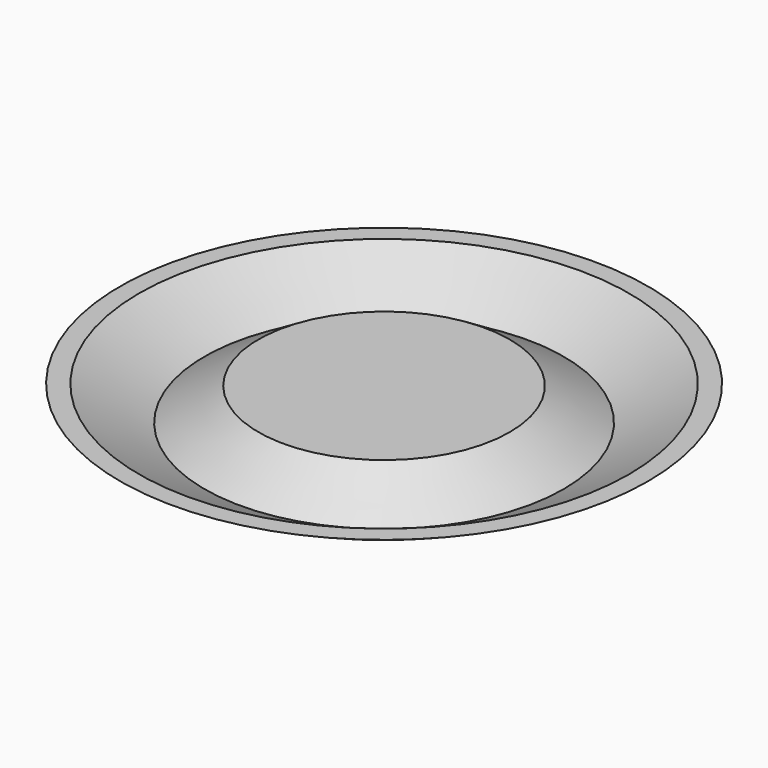
from build123d import *

# Parameters (mm, degrees)
F0_R     = 35
F2_R     = 75
F4_R     = 35
F5_DEPTH = 18
F7_T     = -2.5


# Not quite as in the source:
# - a fillet or chamfer that OpenCascade refuses, or shapes differently, is made with other operations: its cross-section is extruded or revolved along the edge and cut away or added


with BuildPart() as f3:
    # F0 (on Top) → F3 section 0
    with BuildSketch(Plane.XY):
        Circle(F0_R)
    # F2 (on offset) → F3 section 1
    with BuildSketch(Plane.XY.offset(21)):
        Circle(F2_R)
    loft()

    # F4 (on face) → F5 (cut)
    with BuildSketch(Plane(origin=(0, 0, 0), x_dir=(1, 0, 0), z_dir=(0, 0, -1))):
        Circle(F4_R)
    extrude(amount=-F5_DEPTH, mode=Mode.SUBTRACT)

    # F6: chamfer of 18 on 1 edges, made by hand


with BuildPart() as f6_tool2:
    # F6_s3 → F6_t4 (revolve)
    with BuildSketch(Plane.XZ):
        Polygon((50.9371622511, 8.3670101818), (35, 18), (35, 0), align=None)
    revolve(axis=Axis((0, 0, 0), (0, 0, 1)))

    split(bisect_by=Plane.XY.offset(18), keep=Keep.BOTTOM)


with BuildPart() as f3_1:
    add(f3.part)

    # F6_t1: cut F6_tool2
    add(f6_tool2.part, mode=Mode.SUBTRACT)

    # F7
    f7_openings = [f3_1.faces().sort_by_distance(p)[0] for p in [
        (0, 0, 21),
    ]]
    offset(amount=F7_T, openings=f7_openings, kind=Kind.INTERSECTION)


solid = f3_1.part
